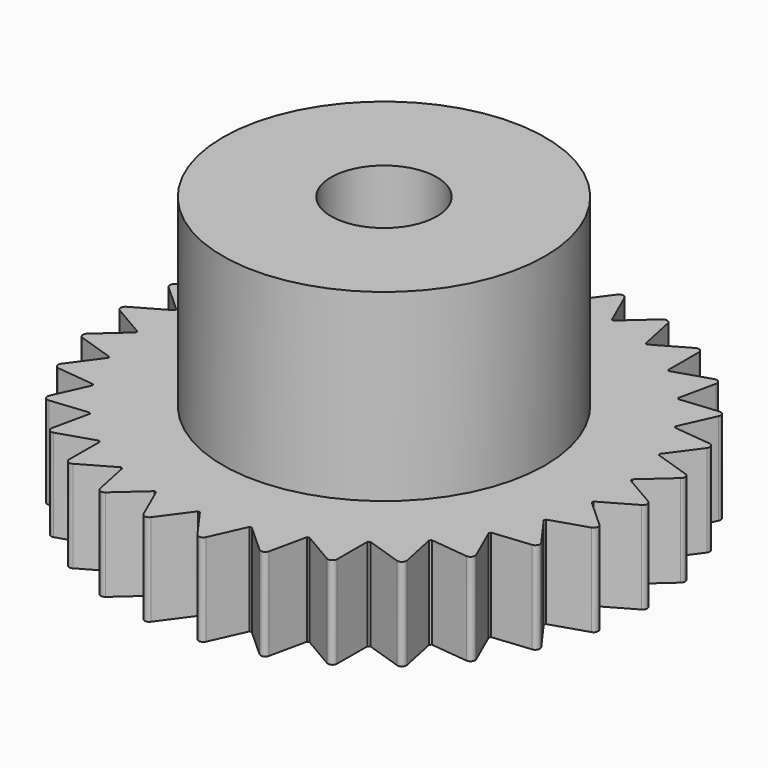
from build123d import *

# Parameters (mm, degrees)
F0_R     = 3.5
F0_R_2   = 1.15
F2_DEPTH = 5
F3_DEPTH = 1
F4_DEPTH = 1
F5_DEPTH = 1
F6_COUNT = 30


with BuildPart() as f2:
    # F0 (on Top) → F2 (new body)
    with BuildSketch(Plane.XY):
        Circle(F0_R)
        Circle(F0_R_2, mode=Mode.SUBTRACT)
    extrude(amount=F2_DEPTH)

    # F0 (on Top) → F3 (join)
    with BuildSketch(Plane.XY):
        Circle(F0_R)
        Circle(F0_R_2, mode=Mode.SUBTRACT)
    extrude(amount=-F3_DEPTH)

    # F0 (on Top) → F4 (join, symmetric)
    with BuildSketch(Plane.XY):
        with BuildLine():
            Line((0, 5), (-0.9949874371, 4.9))
            ThreePointArc((-0.9949874371, 4.9), (0.5, -4.9749371855), (0, 5))
        make_face()
        Circle(F0_R, mode=Mode.SUBTRACT)
    extrude(amount=F4_DEPTH, both=True)

    # F0 (on Top) → F5 (join, symmetric)
    with BuildSketch(Plane.XY):
        with BuildLine():
            Line((-0.6552646986, 5.6537760274), (-0.9949874371, 4.9))
            Line((-0.9949874371, 4.9), (0, 5))
            Line((0, 5), (-0.4829278192, 5.6710965355))
            ThreePointArc((-0.4829278192, 5.6710965355), (-0.5740962589, 5.7121856533), (-0.6552646986, 5.6537760274))
        make_face()
    extrude(amount=F5_DEPTH, both=True)

    # F6: F2 ×30 about axis
    f6_axis = Axis((0, 0, 13.3862942457), (0, 0, 1))


with BuildPart() as f2_1:
    add(f2.part)
    for i in range(1, F6_COUNT):
        add(f2.part.rotate(f6_axis, i * 360 / F6_COUNT))


solid = f2_1.part
